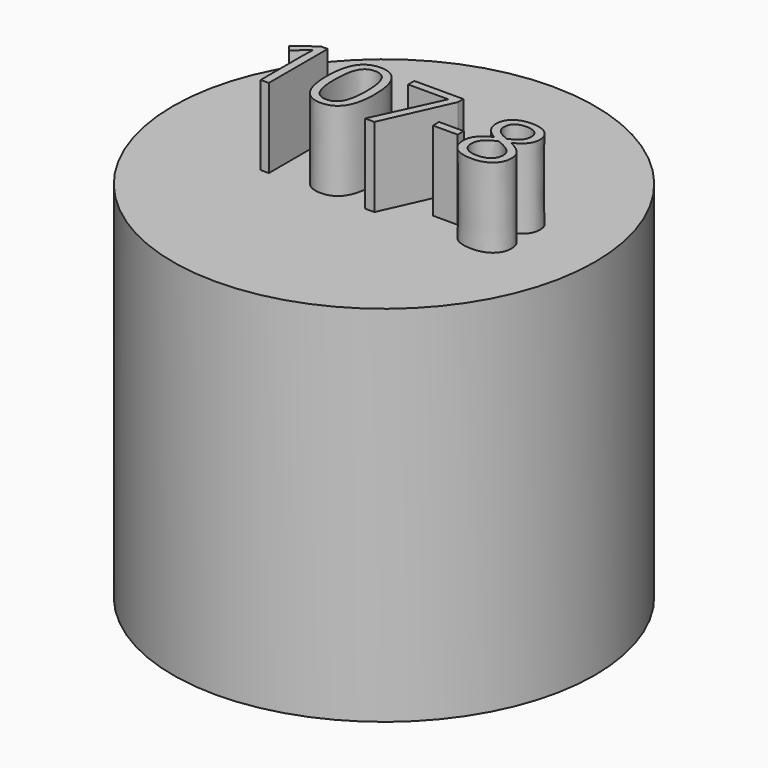
from build123d import *

# Parameters (mm, degrees)
F0_R         = 67.5015485532
F1_DEPTH     = 116.332
F2_TEXT_SIZE = 32.978093562
F3_DEPTH     = 25.4


# Not quite as in the source:
# - Text() gives the source's letters only with a copy of the font that has no kerning and outlines rounded to 1/6400 em; it was checked with that copy


with BuildPart() as f1:
    # F0 (on Top) → F1 (new body)
    with BuildSketch(Plane.XY):
        Circle(F0_R)
    extrude(amount=F1_DEPTH)

    # F2 (on face) → F3 (join)
    with BuildSketch(Plane.XY.offset(116.332)):
        with Locations((-37.6584794722, -13.3614763618)):
            Text('107-8', F2_TEXT_SIZE, font='Open Sans', text_align=(TextAlign.LEFT, TextAlign.BOTTOM))
    extrude(amount=F3_DEPTH)


solid = f1.part
